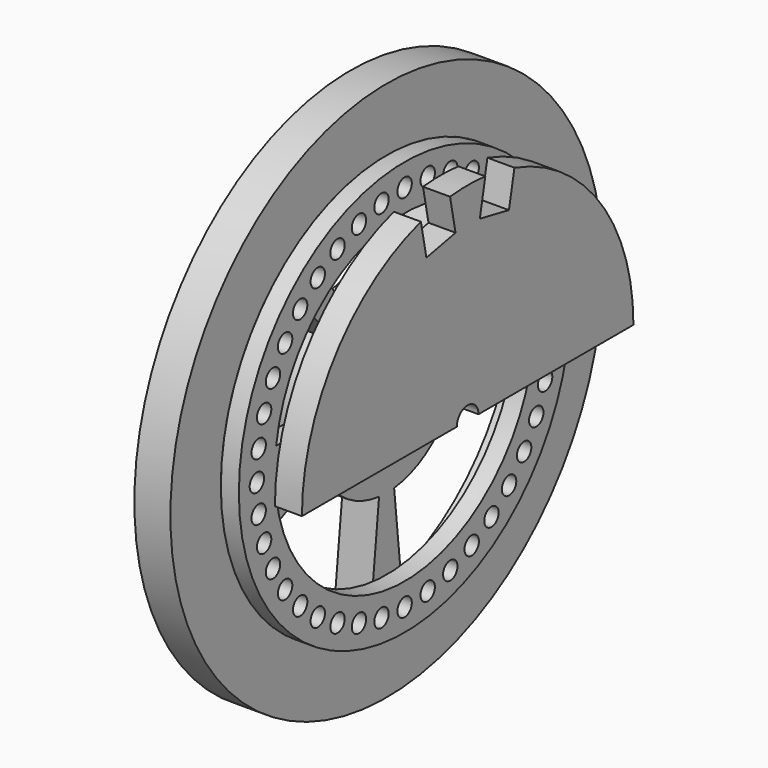
from build123d import *

# Parameters (mm, degrees)
F0_R             = 30
F1_DEPTH         = 4
F2_R             = 3
F3_DEPTH         = 5
F4_R             = 1.25
F4_R_2           = 1.5
F5_DEPTH         = 9.001
F7_DEPTH         = 4.001
F7_COPIES_COUNT  = 5
F8_R             = 23
F8_R_2           = 1.25
F9_DEPTH         = 2
F10_R            = 1
F11_DEPTH        = 6.001
F11_COPIES_COUNT = 40
F14_DEPTH        = 3
F16_DEPTH        = 13.001


# Not quite as in the source:
# - a pattern or mirror of a feature is missing from the dataset's text; its kind, count and spacing are read off the source's solid


with BuildPart() as f1:
    # F0 (on Right) → F1 (new body)
    with BuildSketch(Plane.YZ):
        Circle(F0_R)
    extrude(amount=F1_DEPTH)

    # F2 (on face) → F3 (join)
    with BuildSketch(Plane.YZ.offset(4)):
        Circle(F2_R)
    extrude(amount=F3_DEPTH)

    # F4 (on face) → F5 (cut, through all)
    with BuildSketch(Plane(origin=(0, 0, 0), x_dir=(0, -1, 0), z_dir=(-1, 0, 0))):
        with Locations((-6.35, 0)):
            Circle(F4_R)
        with Locations((6.35, 0)):
            Circle(F4_R)
        Circle(F4_R_2)
    extrude(amount=-F5_DEPTH, mode=Mode.SUBTRACT)

    # F6 (on face) → F7 (cut, through all)
    with BuildSketch(Plane.YZ.offset(4)):
        with BuildLine():
            Line((5, 8.6602540378), (11.5, 19.918584287))
            ThreePointArc((11.5, 19.918584287), (0, 23), (-11.5, 19.918584287))
            Line((-11.5, 19.918584287), (-5, 8.6602540378))
            ThreePointArc((-5, 8.6602540378), (0, 10), (5, 8.6602540378))
        make_face()
    f7 = extrude(amount=-F7_DEPTH, mode=Mode.SUBTRACT)

    # F7_copies: F7 ×5 about axis
    f7_copies_axis = Axis((0, 0, 0), (1, 0, 0))
    for i in range(1, F7_COPIES_COUNT):
        add(f7.rotate(f7_copies_axis, i * 360 / F7_COPIES_COUNT), mode=Mode.SUBTRACT)


with BuildPart() as f9:
    # F8 (on face) → F9 (new body)
    with BuildSketch(Plane.YZ.offset(4)):
        Circle(F8_R)
        with Locations((-6.35, 0)):
            Circle(F8_R_2, mode=Mode.SUBTRACT)
        with BuildLine():
            ThreePointArc((17.82554347, -2.5), (0, -18), (-17.82554347, -2.5))
            Line((-17.82554347, -2.5), (-6.35, -2.5))
            ThreePointArc((-6.35, -2.5), (-3.85, 0), (-6.35, 2.5))
            Line((-6.35, 2.5), (-17.82554347, 2.5))
            ThreePointArc((-17.82554347, 2.5), (0, 18), (17.82554347, 2.5))
            Line((17.82554347, 2.5), (6.35, 2.5))
            ThreePointArc((6.35, 2.5), (3.85, 0), (6.35, -2.5))
            Line((6.35, -2.5), (17.82554347, -2.5))
        make_face(mode=Mode.SUBTRACT)
        with Locations((6.35, 0)):
            Circle(F8_R_2, mode=Mode.SUBTRACT)
    extrude(amount=F9_DEPTH)

    # F10 (on face) → F11 (cut, through all)
    with BuildSketch(Plane.YZ.offset(6)):
        with Locations((0, 20.5)):
            Circle(F10_R)
    f11 = extrude(amount=-F11_DEPTH, mode=Mode.SUBTRACT)

    # F11_copies: F11 ×40 about axis
    f11_copies_axis = Axis((0, 0, 0), (1, 0, 0))
    for i in range(1, F11_COPIES_COUNT):
        add(f11.rotate(f11_copies_axis, i * 360 / F11_COPIES_COUNT), mode=Mode.SUBTRACT)


with BuildPart() as f14:
    # F13 (on offset) → F14 (new body)
    with BuildSketch(Plane.YZ.offset(10)):
        with BuildLine():
            Line((1.5, 0), (23, 0))
            ThreePointArc((23, 0), (0, 23), (-23, 0))
            Line((-23, 0), (-1.5, 0))
            ThreePointArc((-1.5, 0), (0, 1.5), (1.5, 0))
        make_face()
    extrude(amount=F14_DEPTH)

    # F15 (on face) → F16 (cut, through all)
    with BuildSketch(Plane.YZ.offset(13)):
        Polygon((-2.4666597287, 22.9599475126), (-6.507495084, 22.1561753859), (-5.7271337959, 18.2330342643), (-1.6862984407, 19.036806391), align=None)
        Polygon((2.4666597287, 22.9599475126), (1.6862984407, 19.036806391), (5.7271337959, 18.2330342643), (6.507495084, 22.1561753859), align=None)
    extrude(amount=-F16_DEPTH, mode=Mode.SUBTRACT)


solid = Compound([f1.part, f9.part, f14.part])
